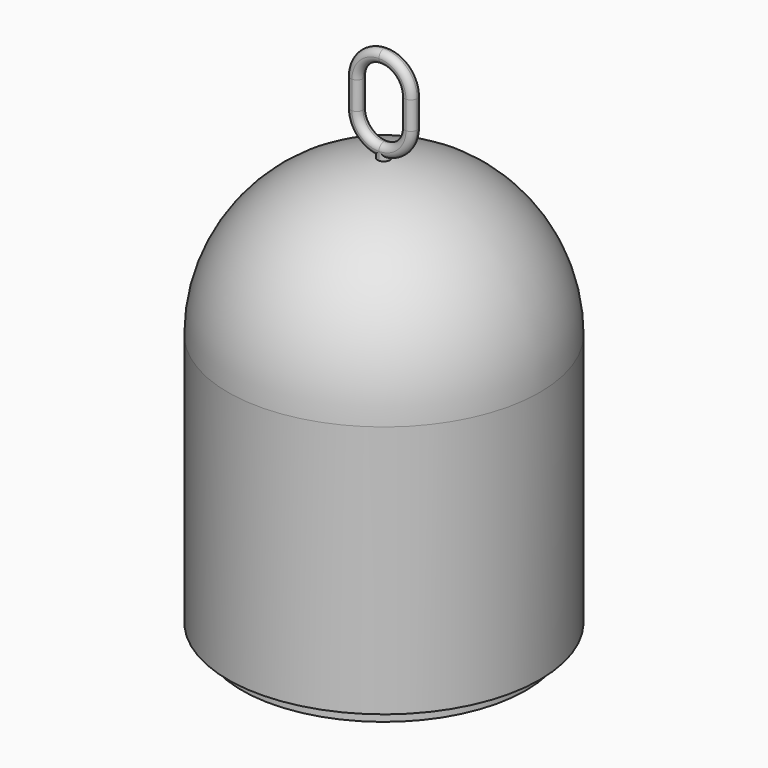
from build123d import *

# Parameters (mm, degrees)
F3_DEPTH      = 0.45
F3_DEPTH_BACK = 0.45
F4_R          = 0.44999


# Not quite as in the source:
# - a fillet or chamfer is up to 0.001 mm smaller than in the source, because OpenCascade refuses the exact size


with BuildPart() as f2:
    # F2: sweep along a path in F1
    with BuildLine(Plane.XY) as f2_path:
        CenterArc((0, 0), 11.25, 0, 360)
    # F0 (on Front) → F2 (sweep)
    with BuildSketch(Plane.XZ):
        with BuildLine():
            Line((0.45, 29.8073129207), (0.45, 29.9909963971))
            ThreePointArc((0.45, 29.9909963971), (0.2250450315, 29.9977488741), (0, 30))
            Line((0, 30), (0, 29.8073129207))
            Line((0, 29.8073129207), (0.45, 29.8073129207))
        make_face()
        with BuildLine():
            Line((11.25, 0.5), (11.25, 18.75))
            ThreePointArc((11.25, 18.75), (8.1124903698, 26.5442286341), (0.45, 29.9909963971))
            Line((0.45, 29.9909963971), (0.45, 29.8073129207))
            Line((0.45, 29.8073129207), (0, 29.8073129207))
            Line((0, 29.8073129207), (0, 29))
            ThreePointArc((0, 29), (7.2478445072, 25.9978445072), (10.25, 18.75))
            Line((10.25, 18.75), (10.25, 1.5))
            Line((10.25, 1.5), (9.25, 1.5))
            Line((9.25, 1.5), (9.25, -0.5))
            Line((9.25, -0.5), (10.25, -0.5))
            Line((10.25, -0.5), (10.25, 0))
            Line((10.25, 0), (10.25, 0.5))
            Line((10.25, 0.5), (11.25, 0.5))
        make_face()
    sweep(path=f2_path.line)

    # F0 (on Front) → F3 (join, two sides)
    with BuildSketch(Plane.XZ) as f3_sk:
        with BuildLine():
            Line((0.45, 29.8073129207), (0.45, 29.9909963971))
            ThreePointArc((0.45, 29.9909963971), (0.2250450315, 29.9977488741), (0, 30))
            Line((0, 30), (0, 29.8073129207))
            Line((0, 29.8073129207), (0.45, 29.8073129207))
        make_face()
        with BuildLine():
            Line((0.45, 30.3073129207), (0.45, 30.1728002437))
            ThreePointArc((0.45, 30.1728002437), (1.8493242009, 31.0005294364), (2.4, 32.5302352905))
            Line((2.4, 32.5302352905), (2.4, 34.5302352905))
            ThreePointArc((2.4, 34.5302352905), (1.6970562748, 36.2272915654), (0, 36.9302352905))
            ThreePointArc((0, 36.9302352905), (-1.6970562748, 36.2272915654), (-2.4, 34.5302352905))
            Line((-2.4, 34.5302352905), (-2.4, 32.5302352905))
            ThreePointArc((-2.4, 32.5302352905), (-1.8493242009, 31.0005294364), (-0.45, 30.1728002437))
            Line((-0.45, 30.1728002437), (-0.45, 30.3073129207))
            Line((-0.45, 30.3073129207), (0.45, 30.3073129207))
        make_face()
        with BuildLine():
            Line((1.5, 34.5302352905), (1.5, 32.5302352905))
            ThreePointArc((1.5, 32.5302352905), (1.0606601718, 31.4695751187), (0, 31.0302352905))
            ThreePointArc((0, 31.0302352905), (-1.0606601718, 31.4695751187), (-1.5, 32.5302352905))
            Line((-1.5, 32.5302352905), (-1.5, 34.5302352905))
            ThreePointArc((-1.5, 34.5302352905), (-1.0606601718, 35.5908954623), (0, 36.0302352905))
            ThreePointArc((0, 36.0302352905), (1.0606601718, 35.5908954623), (1.5, 34.5302352905))
        make_face(mode=Mode.SUBTRACT)
        with BuildLine():
            ThreePointArc((0, 30.1302352905), (0.2260043004, 30.1409002248), (0.45, 30.1728002437))
            Line((0.45, 30.1728002437), (0.45, 30.3073129207))
            Line((0.45, 30.3073129207), (-0.45, 30.3073129207))
            Line((-0.45, 30.3073129207), (-0.45, 30.1728002437))
            ThreePointArc((-0.45, 30.1728002437), (-0.2260043004, 30.1409002248), (0, 30.1302352905))
        make_face()
        with BuildLine():
            ThreePointArc((0, 30), (0.2250450315, 29.9977488741), (0.45, 29.9909963971))
            Line((0.45, 29.9909963971), (0.45, 30.1728002437))
            ThreePointArc((0.45, 30.1728002437), (0.2260043004, 30.1409002248), (0, 30.1302352905))
            ThreePointArc((0, 30.1302352905), (-0.2260043004, 30.1409002248), (-0.45, 30.1728002437))
            Line((-0.45, 30.1728002437), (-0.45, 29.8073129207))
            Line((-0.45, 29.8073129207), (0, 29.8073129207))
            Line((0, 29.8073129207), (0, 30))
        make_face()
    extrude(amount=F3_DEPTH)
    extrude(f3_sk.sketch, amount=-F3_DEPTH_BACK)

    # F4 (radius 0.45 in the source; OpenCascade refuses exactly that, so slightly less here)
    f4_edges = [f2.edges().sort_by_distance(p)[0] for p in [
        (0, -0.45, 31.030235),
        (0, 0.45, 31.030235),
        (0, -0.45, 36.930235),
        (0, 0.45, 36.930235),
        (0.45, -0.45, 30.077393),
        (0.45, 0.45, 30.077393),
        (-0.45, -0.45, 30.077393),
        (-0.45, 0.45, 30.077393),
        (-1.849324, 0.45, 31.000529),
        (-2.4, 0.45, 33.530235),
        (2.4, 0.45, 33.530235),
        (1.849324, 0.45, 31.000529),
        (1.5, 0.45, 33.530235),
        (-1.5, 0.45, 33.530235),
        (0, 0.45, 36.030235),
        (-1.849324, -0.45, 31.000529),
        (-2.4, -0.45, 33.530235),
        (2.4, -0.45, 33.530235),
        (1.849324, -0.45, 31.000529),
        (1.5, -0.45, 33.530235),
        (-1.5, -0.45, 33.530235),
        (0, -0.45, 36.030235),
    ]]
    fillet(f4_edges, radius=F4_R)


solid = f2.part
